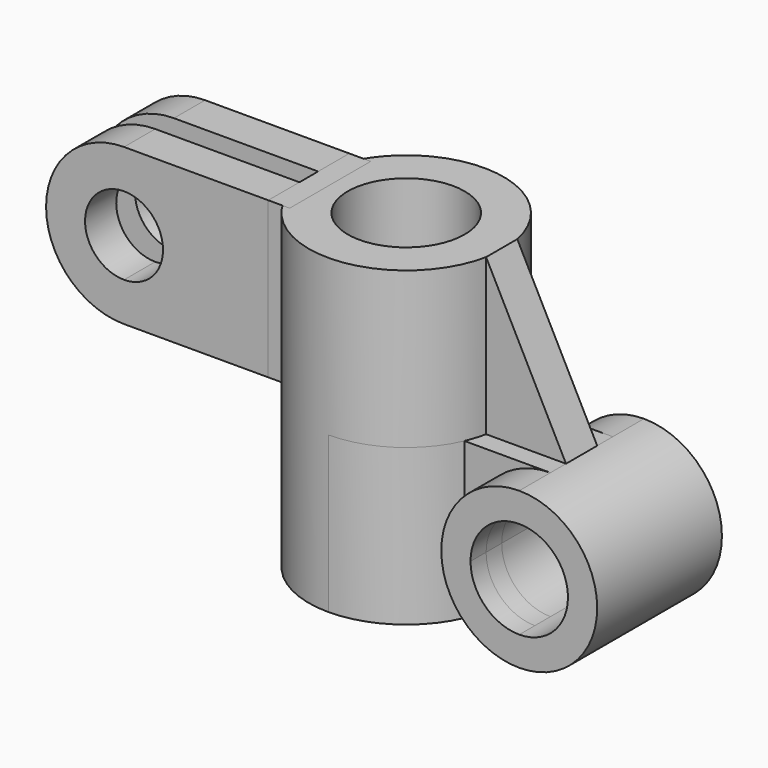
from build123d import *

# Parameters (mm, degrees)
F0_R           = 25
F0_R_2         = 15
F1_DEPTH       = 80
F4_DEPTH       = 40
F6_DEPTH       = 25
F7_R           = 15
F8_DEPTH       = 40
F10_DEPTH      = 49.5
F12_DEPTH      = 10
F12_DEPTH_BACK = 30
F13_DEPTH      = 25
F17_DEPTH      = 13
F17_DEPTH_BACK = 13
F18_W          = 26
F18_H          = 40
F19_DEPTH      = 5.5
F20_W          = 37
F20_H          = 3
F21_DEPTH      = 156.4


with BuildPart() as f1:
    # F0 (on Top) → F1 (new body)
    with BuildSketch(Plane.XY):
        Circle(F0_R)
        Circle(F0_R_2, mode=Mode.SUBTRACT)
    extrude(amount=F1_DEPTH)

    # F3 (on face) → F4 (join)
    with BuildSketch(Plane.XY.offset(80)):
        with BuildLine():
            ThreePointArc((24.4948974278, 5), (24.8734038251, 2.5127240501), (25, 0))
            Line((25, 0), (45, 0))
            Line((45, 0), (45, 5))
            Line((45, 5), (24.4948974278, 5))
        make_face()
        with BuildLine():
            Line((45, 0), (25, 0))
            ThreePointArc((25, 0), (24.8734038251, -2.5127240501), (24.4948974278, -5))
            Line((24.4948974278, -5), (45, -5))
            Line((45, -5), (45, 0))
        make_face()
    extrude(amount=-F4_DEPTH)

    # F5 (on face) → F6 (cut)
    with BuildSketch(Plane.XZ.offset(5)):
        Polygon((45, 80), (24.4948974278, 80), (45, 40), align=None)
    extrude(amount=-F6_DEPTH, mode=Mode.SUBTRACT)

    # F7 (on Top) → F8 (join)
    with BuildSketch(Plane.XY):
        with BuildLine():
            ThreePointArc((0, -25), (17.6776695297, -17.6776695297), (25, 0))
            ThreePointArc((25, 0), (17.6776695297, 17.6776695297), (0, 25))
            ThreePointArc((0, 25), (-25, 0), (0, -25))
        make_face()
        Circle(F7_R, mode=Mode.SUBTRACT)
        with BuildLine():
            ThreePointArc((0, 25), (17.6776695297, 17.6776695297), (25, 0))
            ThreePointArc((25, 0), (17.6776695297, -17.6776695297), (0, -25))
            Line((0, -25), (57, -25))
            Line((57, -25), (57, 25))
            Line((57, 25), (0, 25))
        make_face()
    extrude(amount=F8_DEPTH)

    # F9 (on face) → F10 (cut)
    with BuildSketch(Plane.XY.offset(40)):
        with BuildLine():
            Line((45, 5), (45, 0))
            Line((45, 0), (45, -5))
            Line((45, -5), (45, -10))
            Line((45, -10), (22.9128784748, -10))
            ThreePointArc((22.9128784748, -10), (13.6930639376, -20.9165006634), (0, -25))
            Line((0, -25), (57, -25))
            Line((57, -25), (57, 25))
            Line((57, 25), (0, 25))
            ThreePointArc((0, 25), (13.6930639376, 20.9165006634), (22.9128784748, 10))
            Line((22.9128784748, 10), (24.4948974278, 10))
            Line((24.4948974278, 10), (45, 10))
            Line((45, 10), (45, 5))
        make_face()
    extrude(amount=-F10_DEPTH, mode=Mode.SUBTRACT)

    # F11 (on face) → F12 (join, two sides)
    with BuildSketch(Plane(origin=(0, 10, 0), x_dir=(-1, 0, 0), z_dir=(0, 1, 0))) as f12_sk:
        with BuildLine():
            ThreePointArc((-45, 0), (-30.8578643763, 5.8578643763), (-25, 20))
            ThreePointArc((-25, 20), (-30.8578643763, 34.1421356237), (-45, 40))
            Line((-45, 40), (-45, 32.5))
            ThreePointArc((-45, 32.5), (-36.1611652352, 28.8388347648), (-32.5, 20))
            ThreePointArc((-32.5, 20), (-36.1611652352, 11.1611652352), (-45, 7.5))
            Line((-45, 7.5), (-45, 0))
        make_face()
        with BuildLine():
            Line((-45, 32.5), (-45, 40))
            ThreePointArc((-45, 40), (-65, 20), (-45, 0))
            Line((-45, 0), (-45, 7.5))
            ThreePointArc((-45, 7.5), (-57.5, 20), (-45, 32.5))
        make_face()
    extrude(amount=F12_DEPTH)
    extrude(f12_sk.sketch, amount=-F12_DEPTH_BACK)

    # F13 (cut): a face of the model
    f13_faces = [f1.faces().sort_by_distance(p)[0] for p in [
        (39.6948352303, 10, 20),
    ]]
    extrude(f13_faces, amount=-F13_DEPTH, mode=Mode.SUBTRACT)


with BuildPart() as f17:
    # F16 (on Front) → F17 (new body, two sides)
    with BuildSketch(Plane.XZ) as f17_sk:
        with BuildLine():
            Line((-25, 40), (-25, 80))
            Line((-25, 80), (-62, 80))
            ThreePointArc((-62, 80), (-47.8578643763, 74.1421356237), (-42, 60))
            ThreePointArc((-42, 60), (-47.8578643763, 45.8578643763), (-62, 40))
            Line((-62, 40), (-25, 40))
        make_face()
        with BuildLine():
            ThreePointArc((-42, 60), (-47.8578643763, 74.1421356237), (-62, 80))
            Line((-62, 80), (-62, 70))
            ThreePointArc((-62, 70), (-54.9289321881, 67.0710678119), (-52, 60))
            ThreePointArc((-52, 60), (-54.9289321881, 52.9289321881), (-62, 50))
            Line((-62, 50), (-62, 40))
            ThreePointArc((-62, 40), (-47.8578643763, 45.8578643763), (-42, 60))
        make_face()
        with BuildLine():
            Line((-62, 70), (-62, 80))
            ThreePointArc((-62, 80), (-82, 60), (-62, 40))
            Line((-62, 40), (-62, 50))
            ThreePointArc((-62, 50), (-72, 60), (-62, 70))
        make_face()
    extrude(amount=F17_DEPTH)
    extrude(f17_sk.sketch, amount=-F17_DEPTH_BACK)

    # F20 (on face) → F21 (cut)
    with BuildSketch(Plane.XY.offset(80)):
        with Locations((-43.5, 1.5)):
            Rectangle(F20_W, F20_H)
        with Locations((-43.5, -1.5)):
            Rectangle(F20_W, F20_H)
        Polygon((-62, -3), (-62, 0), (-62, 3), (-82, 3), (-82, -3), align=None)
    extrude(amount=-F21_DEPTH, mode=Mode.SUBTRACT)


with BuildPart() as f19:
    # F18 (on face) → F19 (new body)
    with BuildSketch(Plane.YZ.offset(-25)):
        with Locations((0, 60)):
            Rectangle(F18_W, F18_H)
    extrude(amount=F19_DEPTH)


solid = Compound([f1.part, f17.part, f19.part])
